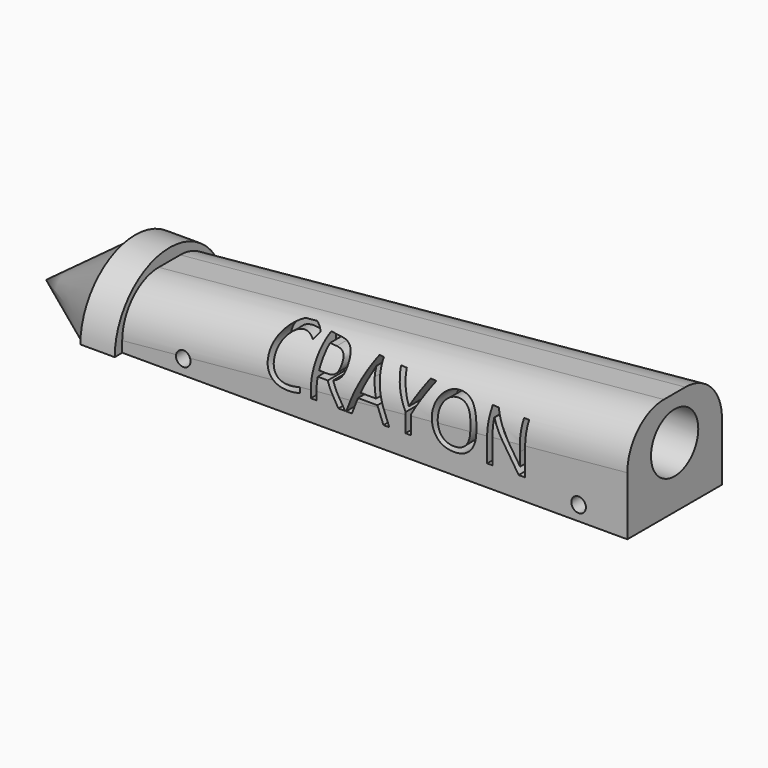
from build123d import *

# Parameters (mm, degrees)
F3_DEPTH       = 19.05
F3_DEPTH_BACK  = 19.05
F4_R           = 14.7170458762
F6_TEXT_SIZE   = 21.9477010736
F7_DEPTH       = 10.16
F8_R           = 2.3451033347
F8_R_2         = 2.3613313818
F9_DEPTH       = 25.4
F9_DEPTH_BACK  = 25.4
F10_R          = 9.525
F11_DEPTH      = 25.4
F5_W           = 220.2693223953
F5_H           = 25.8888117969
F12_DEPTH      = 25.4
F12_DEPTH_BACK = 25.4
F13_ANGLE_BACK = 90
F13_ANGLE      = 180
F14_ANGLE_BACK = 90
F14_ANGLE      = 180


# Not quite as in the source:
# - Text() gives the source's letters only with a copy of the font that has no kerning and outlines rounded to 1/6400 em; it was checked with that copy


with BuildPart() as f3:
    # F0 (on Front) → F3 (new body, two sides)
    with BuildSketch(Plane.XZ) as f3_sk:
        Polygon((-74.111096561, 18.0295741786), (-74.111096561, 0), (90.988903439, 0), (90.988903439, 33.6862241155), align=None)
    extrude(amount=F3_DEPTH)
    extrude(f3_sk.sketch, amount=-F3_DEPTH_BACK)

    # F4
    f4_edges = [f3.edges().sort_by_distance(p)[0] for p in [
        (8.438903, -19.05, 25.857899),
        (8.438903, 19.05, 25.857899),
    ]]
    fillet(f4_edges, radius=F4_R)

    # F6 (on face) → F7 (cut)
    with BuildSketch(Plane.XZ.offset(19.05)):
        with Locations((-27.0344316959, 6.8499795161)):
            Text('CRAYON', F6_TEXT_SIZE, font='Open Sans', text_align=(TextAlign.LEFT, TextAlign.BOTTOM))
    extrude(amount=-F7_DEPTH, mode=Mode.SUBTRACT)

    # F8 (on Front) → F9 (cut, two sides)
    with BuildSketch(Plane.XZ) as f9_sk:
        with Locations((-52.1348230541, 4.698342178)):
            Circle(F8_R)
        with Locations((75.2731561661, 4.698342178)):
            Circle(F8_R_2)
    extrude(amount=F9_DEPTH, mode=Mode.SUBTRACT)
    extrude(f9_sk.sketch, amount=-F9_DEPTH_BACK, mode=Mode.SUBTRACT)

    # F10 (on face) → F11 (cut)
    with BuildSketch(Plane.YZ.offset(90.988903439)):
        with Locations((0, 19.685)):
            Circle(F10_R)
    extrude(amount=-F11_DEPTH, mode=Mode.SUBTRACT)

    # F5 (on Front) → F12 (cut, two sides)
    with BuildSketch(Plane.XZ) as f12_sk:
        with Locations((-4.7368407249, -12.9444058985)):
            Rectangle(F5_W, F5_H)
    extrude(amount=-F12_DEPTH, mode=Mode.SUBTRACT)
    extrude(f12_sk.sketch, amount=F12_DEPTH_BACK, mode=Mode.SUBTRACT)



with BuildPart() as f13:
    # F2 (on Front) → F13 (revolve)
    with BuildSketch(Plane.XZ, mode=Mode.PRIVATE) as f13_sk:
        Polygon((-82.8451290727, 0), (-83.1215009093, 21.0043527186), (-111.5879267454, 0), align=None)
    revolve(f13_sk.sketch.rotate(Axis((-97.216527909, 0, 0), (1, 0, 0)), -F13_ANGLE_BACK), axis=Axis((-97.216527909, 0, 0), (1, 0, 0)), revolution_arc=F13_ANGLE)


with BuildPart() as f3_1:
    add(f3.part)

    add(f13.part)  # F14 merges F13
    # F1 (on Front) → F14 (revolve)
    with BuildSketch(Plane.XZ, mode=Mode.PRIVATE) as f14_sk:
        Polygon((-72.0665827394, 0), (-71.7717013578, 22.1162009984), (-82.8451290727, 22.1162009984), (-82.8451290727, 0), align=None)
    revolve(f14_sk.sketch.rotate(Axis((-77.455855906, 0, 0), (1, 0, 0)), -F14_ANGLE_BACK), axis=Axis((-77.455855906, 0, 0), (1, 0, 0)), revolution_arc=F14_ANGLE)


solid = f3_1.part
